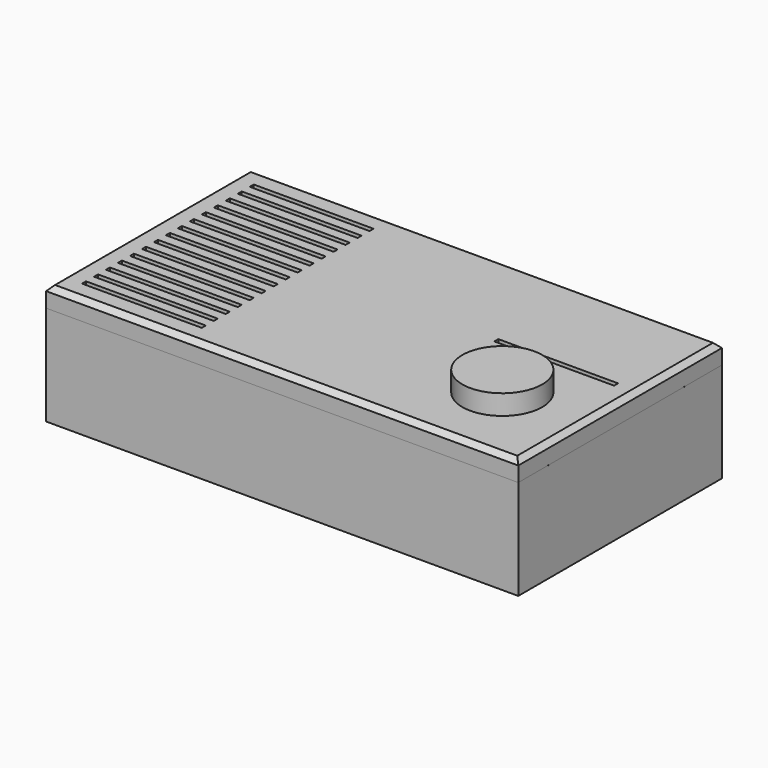
from build123d import *

# Parameters (mm, degrees)
F1_W      = 20
F1_H      = 255
F2_DEPTH  = 100
F3_DEPTH  = 100
F0_W      = 473
F0_H      = 20
F4_DEPTH  = 100
F5_DEPTH  = 100
F6_SIZE   = 19.99999
F7_SIZE   = 19.99999
F8_SIZE   = 19.99999
F9_SIZE   = 19.99999
F10_W     = 473
F10_H     = 255
F11_DEPTH = 20
F13_SIZE  = 5
F14_W     = 120
F14_H     = 5
F15_DEPTH = 10
F19_R     = 40
F20_DEPTH = 20


# Not quite as in the source:
# - a fillet or chamfer is up to 0.001 mm smaller than in the source, because OpenCascade refuses the exact size


with BuildPart() as f2:
    # F1 (on Top) → F2 (new body)
    with BuildSketch(Plane.XY):
        with Locations((-226.5, 0)):
            Rectangle(F1_W, F1_H)
    extrude(amount=F2_DEPTH)

    # F6 (size 20 in the source; OpenCascade refuses exactly that, so slightly less here)
    f6_edges = [f2.edges().sort_by_distance(p)[0] for p in [
        (-216.5, -127.5, 50),
        (-216.5, 127.5, 50),
    ]]
    chamfer(f6_edges, length=F6_SIZE)


with BuildPart() as f3:
    # F1 (on Top) → F3 (new body)
    with BuildSketch(Plane.XY):
        with Locations((226.5022045374, 0)):
            Rectangle(F1_W, F1_H)
    extrude(amount=F3_DEPTH)

    # F7 (size 20 in the source; OpenCascade refuses exactly that, so slightly less here)
    f7_edges = [f3.edges().sort_by_distance(p)[0] for p in [
        (216.502205, -127.5, 50),
        (216.502205, 127.5, 50),
    ]]
    chamfer(f7_edges, length=F7_SIZE)


with BuildPart() as f4:
    # F0 (on Top) → F4 (new body)
    with BuildSketch(Plane.XY):
        with Locations((0, -117.5)):
            Rectangle(F0_W, F0_H)
    extrude(amount=F4_DEPTH)

    # F8 (size 20 in the source; OpenCascade refuses exactly that, so slightly less here)
    f8_edges = [f4.edges().sort_by_distance(p)[0] for p in [
        (236.5, -107.5, 50),
        (-236.5, -107.5, 50),
    ]]
    chamfer(f8_edges, length=F8_SIZE)


with BuildPart() as f5:
    # F0 (on Top) → F5 (new body)
    with BuildSketch(Plane.XY):
        with Locations((0, 117.5)):
            Rectangle(F0_W, F0_H)
    extrude(amount=F5_DEPTH)

    # F9 (size 20 in the source; OpenCascade refuses exactly that, so slightly less here)
    f9_edges = [f5.edges().sort_by_distance(p)[0] for p in [
        (-236.5, 107.5, 50),
        (236.5, 107.5, 50),
    ]]
    chamfer(f9_edges, length=F9_SIZE)


with BuildPart() as f11:
    # F10 (on Top) → F11 (new body)
    with BuildSketch(Plane.XY):
        Rectangle(F10_W, F10_H)
    extrude(amount=F11_DEPTH)


with BuildPart() as f11_1:
    # F12: moved
    add(f11.part.moved(Location((0, 0, 100))))

    # F13
    f13_edges = [f11_1.edges().sort_by_distance(p)[0] for p in [
        (0, -127.5, 120),
        (236.5, 0, 120),
        (0, 127.5, 120),
        (-236.5, 0, 120),
    ]]
    chamfer(f13_edges, length=F13_SIZE)


with BuildPart() as f15:
    # F14 (on Top) → F15 (new body)
    with BuildSketch(Plane.XY):
        with Locations((-156.5, 105)):
            Rectangle(F14_W, F14_H)
    extrude(amount=-F15_DEPTH)


with BuildPart() as f15b:
    # F14 (on Top) → F15, piece 2 (new body)
    with BuildSketch(Plane.XY):
        with Locations((-156.4999991655, 90)):
            Rectangle(F14_W, F14_H)
    extrude(amount=-F15_DEPTH)


with BuildPart() as f15c:
    # F14 (on Top) → F15, piece 3 (new body)
    with BuildSketch(Plane.XY):
        with Locations((-156.5, 75)):
            Rectangle(F14_W, F14_H)
    extrude(amount=-F15_DEPTH)


with BuildPart() as f15d:
    # F14 (on Top) → F15, piece 4 (new body)
    with BuildSketch(Plane.XY):
        with Locations((-156.4999991655, 60)):
            Rectangle(F14_W, F14_H)
    extrude(amount=-F15_DEPTH)


with BuildPart() as f15e:
    # F14 (on Top) → F15, piece 5 (new body)
    with BuildSketch(Plane.XY):
        with Locations((-156.5, 45)):
            Rectangle(F14_W, F14_H)
    extrude(amount=-F15_DEPTH)


with BuildPart() as f15f:
    # F14 (on Top) → F15, piece 6 (new body)
    with BuildSketch(Plane.XY):
        with Locations((-156.4999991655, 30)):
            Rectangle(F14_W, F14_H)
    extrude(amount=-F15_DEPTH)


with BuildPart() as f15g:
    # F14 (on Top) → F15, piece 7 (new body)
    with BuildSketch(Plane.XY):
        with Locations((-156.5, 15)):
            Rectangle(F14_W, F14_H)
    extrude(amount=-F15_DEPTH)


with BuildPart() as f15h:
    # F14 (on Top) → F15, piece 8 (new body)
    with BuildSketch(Plane.XY):
        with Locations((-156.4999991655, 0)):
            Rectangle(F14_W, F14_H)
    extrude(amount=-F15_DEPTH)


with BuildPart() as f15i:
    # F14 (on Top) → F15, piece 9 (new body)
    with BuildSketch(Plane.XY):
        with Locations((-156.5, -15)):
            Rectangle(F14_W, F14_H)
    extrude(amount=-F15_DEPTH)


with BuildPart() as f15j:
    # F14 (on Top) → F15, piece 10 (new body)
    with BuildSketch(Plane.XY):
        with Locations((-156.4999991655, -30)):
            Rectangle(F14_W, F14_H)
    extrude(amount=-F15_DEPTH)


with BuildPart() as f15k:
    # F14 (on Top) → F15, piece 11 (new body)
    with BuildSketch(Plane.XY):
        with Locations((-156.5, -45)):
            Rectangle(F14_W, F14_H)
    extrude(amount=-F15_DEPTH)


with BuildPart() as f15l:
    # F14 (on Top) → F15, piece 12 (new body)
    with BuildSketch(Plane.XY):
        with Locations((-156.4999991655, -60)):
            Rectangle(F14_W, F14_H)
    extrude(amount=-F15_DEPTH)


with BuildPart() as f15m:
    # F14 (on Top) → F15, piece 13 (new body)
    with BuildSketch(Plane.XY):
        with Locations((-156.5, -75)):
            Rectangle(F14_W, F14_H)
    extrude(amount=-F15_DEPTH)


with BuildPart() as f15n:
    # F14 (on Top) → F15, piece 14 (new body)
    with BuildSketch(Plane.XY):
        with Locations((-156.4999991655, -90)):
            Rectangle(F14_W, F14_H)
    extrude(amount=-F15_DEPTH)


with BuildPart() as f15o:
    # F14 (on Top) → F15, piece 15 (new body)
    with BuildSketch(Plane.XY):
        with Locations((-156.5, -105)):
            Rectangle(F14_W, F14_H)
    extrude(amount=-F15_DEPTH)


with BuildPart() as f15p:
    # F14 (on Top) → F15, piece 16 (new body)
    with BuildSketch(Plane.XY):
        with Locations((-16.4999985695, 0)):
            Rectangle(F14_W, F14_H)
    extrude(amount=-F15_DEPTH)


with BuildPart() as f15o_1:
    # F16: moved
    add(f15o.part.moved(Location((0, 0, 120))))


with BuildPart() as f15n_1:
    # F16: moved
    add(f15n.part.moved(Location((0, 0, 120))))


with BuildPart() as f15m_1:
    # F16: moved
    add(f15m.part.moved(Location((0, 0, 120))))


with BuildPart() as f15l_1:
    # F16: moved
    add(f15l.part.moved(Location((0, 0, 120))))


with BuildPart() as f15k_1:
    # F16: moved
    add(f15k.part.moved(Location((0, 0, 120))))


with BuildPart() as f15j_1:
    # F16: moved
    add(f15j.part.moved(Location((0, 0, 120))))


with BuildPart() as f15e_1:
    # F16: moved
    add(f15e.part.moved(Location((0, 0, 120))))


with BuildPart() as f15f_1:
    # F16: moved
    add(f15f.part.moved(Location((0, 0, 120))))


with BuildPart() as f15g_1:
    # F16: moved
    add(f15g.part.moved(Location((0, 0, 120))))


with BuildPart() as f15h_1:
    # F16: moved
    add(f15h.part.moved(Location((0, 0, 120))))


with BuildPart() as f15i_1:
    # F16: moved
    add(f15i.part.moved(Location((0, 0, 120))))


with BuildPart() as f15_1:
    # F16: moved
    add(f15.part.moved(Location((0, 0, 120))))


with BuildPart() as f15b_1:
    # F16: moved
    add(f15b.part.moved(Location((0, 0, 120))))


with BuildPart() as f15c_1:
    # F16: moved
    add(f15c.part.moved(Location((0, 0, 120))))


with BuildPart() as f15d_1:
    # F16: moved
    add(f15d.part.moved(Location((0, 0, 120))))


with BuildPart() as f15p_1:
    # F16: moved
    add(f15p.part.moved(Location((0, 0, 120))))


with BuildPart() as f15p_2:
    # F17: moved
    add(f15p_1.part.moved(Location((173, 20, 0))))


with BuildPart() as f11_2:
    add(f11_1.part)

    # F18: cut F15o, F15n, F15m, F15l, F15k, F15j, F15i, F15c, F15d, F15e, F15f, F15g, F15h, F15, F15b, F15p
    add(f15o_1.part, mode=Mode.SUBTRACT)
    add(f15n_1.part, mode=Mode.SUBTRACT)
    add(f15m_1.part, mode=Mode.SUBTRACT)
    add(f15l_1.part, mode=Mode.SUBTRACT)
    add(f15k_1.part, mode=Mode.SUBTRACT)
    add(f15j_1.part, mode=Mode.SUBTRACT)
    add(f15i_1.part, mode=Mode.SUBTRACT)
    add(f15c_1.part, mode=Mode.SUBTRACT)
    add(f15d_1.part, mode=Mode.SUBTRACT)
    add(f15e_1.part, mode=Mode.SUBTRACT)
    add(f15f_1.part, mode=Mode.SUBTRACT)
    add(f15g_1.part, mode=Mode.SUBTRACT)
    add(f15h_1.part, mode=Mode.SUBTRACT)
    add(f15_1.part, mode=Mode.SUBTRACT)
    add(f15b_1.part, mode=Mode.SUBTRACT)
    add(f15p_2.part, mode=Mode.SUBTRACT)


with BuildPart() as f20:
    # F19 (on Top) → F20 (new body)
    with BuildSketch(Plane.XY):
        with Locations((156.5022045374, -47.5)):
            Circle(F19_R)
    extrude(amount=F20_DEPTH)


with BuildPart() as f20_1:
    # F21: moved
    add(f20.part.moved(Location((0, 0, 121))))


solid = Compound([f2.part, f3.part, f4.part, f5.part, f11_2.part, f20_1.part])
